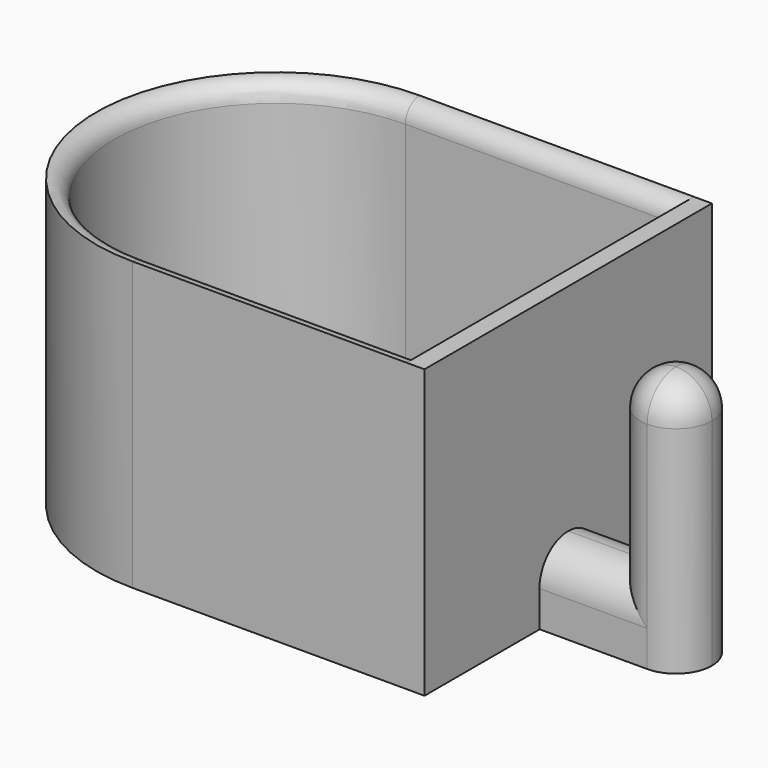
from build123d import *

# Parameters (mm, degrees)
F1_DEPTH = 40
F2_T     = -2.5
F3_W     = 10
F3_H     = 10
F4_DEPTH = 20
F5_W     = 10
F5_H     = 10
F6_DEPTH = 25
F7_R     = 4.99999
F8_R     = 2.49999


# Not quite as in the source:
# - a fillet or chamfer is up to 0.001 mm smaller than in the source, because OpenCascade refuses the exact size


with BuildPart() as f1:
    # F0 (on Top) → F1 (new body)
    with BuildSketch(Plane.XY):
        with BuildLine():
            Line((40.6640707215, 25), (0, 25))
            ThreePointArc((0, 25), (-25, 0), (0, -25))
            Line((0, -25), (40.6640707215, -25))
            Line((40.6640707215, -25), (40.6640707215, 25))
        make_face()
    extrude(amount=F1_DEPTH)

    # F2
    f2_openings = [f1.faces().sort_by_distance(p)[0] for p in [
        (10.256385, 0, 40),
    ]]
    offset(amount=F2_T, openings=f2_openings)

    # F3 (on face) → F4 (join)
    with BuildSketch(Plane.YZ.offset(40.6640707215)):
        with Locations((0, 5.0200799115)):
            Rectangle(F3_W, F3_H)
    extrude(amount=F4_DEPTH)

    # F5 (on face) → F6 (join)
    with BuildSketch(Plane.XY.offset(10.0200799115)):
        with Locations((55.6640707215, 0)):
            Rectangle(F5_W, F5_H)
    extrude(amount=F6_DEPTH)

    # F7 (radius 5 in the source; OpenCascade refuses exactly that, so slightly less here)
    f7_edges = [f1.edges().sort_by_distance(p)[0] for p in [
        (45.664071, -5, 10.02008),
        (45.664071, 5, 10.02008),
        (50.664071, -5, 22.52008),
        (50.664071, 5, 22.52008),
        (55.664071, -5, 35.02008),
        (60.664071, 0, 35.02008),
        (55.664071, 5, 35.02008),
        (50.664071, 0, 35.02008),
        (60.664071, -5, 17.52008),
        (60.664071, 5, 17.52008),
    ]]
    fillet(f7_edges, radius=F7_R)

    # F8 (radius 2.5 in the source; OpenCascade refuses exactly that, so slightly less here)
    f8_edges = [f1.edges().sort_by_distance(p)[0] for p in [
        (-22.5, 0, 40),
    ]]
    fillet(f8_edges, radius=F8_R)


solid = f1.part
